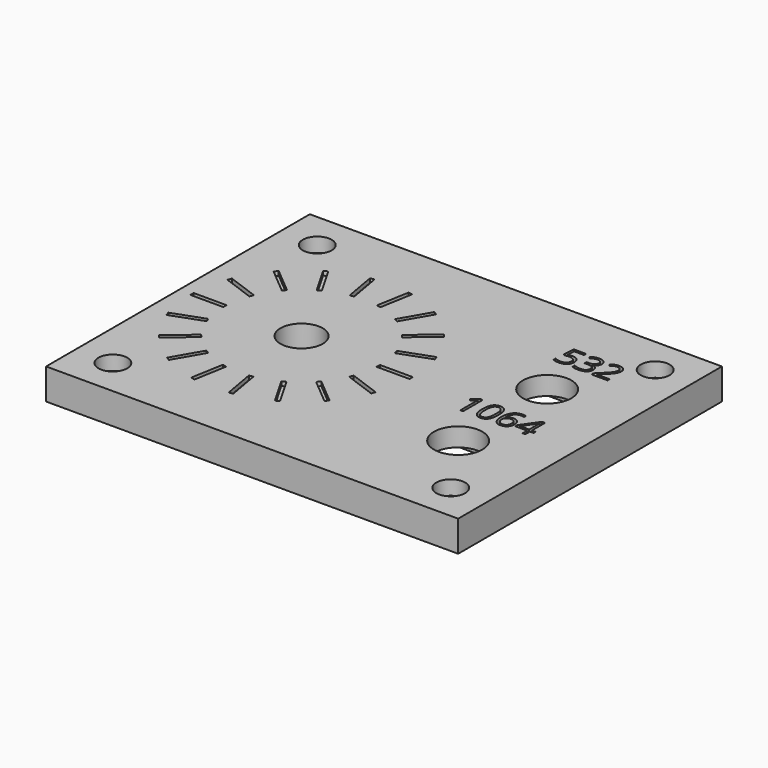
from build123d import *

# Parameters (mm, degrees)
F0_W          = 100
F0_H          = 80
F1_DEPTH      = 6
F2_R          = 5.125
F3_DEPTH      = 25
F4_W          = 8
F4_H          = 1
F5_DEPTH      = 1
F6_R          = 5.875
F7_DEPTH      = 6.001
F8_W          = 25
F8_H          = 14
F9_DEPTH      = 1.5
F10_R         = 3.5
F11_DEPTH     = 3.5
F12_R         = 2.375
F13_DEPTH     = 6.001
F14_TEXT_SIZE = 8.3333333333
F15_DEPTH     = 1.5
F16_W         = 100
F16_H         = 80
F16_W_2       = 96
F16_H_2       = 76
F17_DEPTH     = 1.5
F18_W         = 4
F18_H         = 4
F19_DEPTH     = 3


# Not quite as in the source:
# - Text() gives the source's letters only with a copy of the font that has no kerning and outlines rounded to 1/6400 em; it was checked with that copy


with BuildPart() as f1:
    # F0 (on Top) → F1 (new body)
    with BuildSketch(Plane.XY):
        with Locations((50, 40)):
            Rectangle(F0_W, F0_H)
    extrude(amount=F1_DEPTH)

    # F2 (on face) → F3 (cut)
    with BuildSketch(Plane.XY.offset(6)):
        with Locations((30, 40)):
            Circle(F2_R)
    extrude(amount=-F3_DEPTH, mode=Mode.SUBTRACT)

    # F4 (on face) → F5 (cut)
    with BuildSketch(Plane.XY.offset(6)):
        with Locations((7, 40.5)):
            Rectangle(F4_W, F4_H)
        Polygon((4.6282992388, 30.7654561302), (12.1458402051, 33.5016172768), (11.8038200617, 34.4413098976), (4.2862790955, 31.705148751), align=None)
        Polygon((9.3168000358, 22.6447345385), (15.4451555807, 27.787035416), (14.8023679711, 28.5530798591), (8.6740124261, 23.4107789816), align=None)
        Polygon((16.5, 16.6173140978), (20.5, 23.5455173281), (19.6339745962, 24.0455173281), (15.6339745962, 17.1173140978), align=None)
        Polygon((25.311499203, 13.4101906687), (26.7006846243, 21.2886526928), (25.7158768713, 21.4623008704), (24.32669145, 13.5838388463), align=None)
        Polygon((34.688500797, 13.4101906687), (33.2993153757, 21.2886526928), (32.3145076227, 21.1150045151), (33.703693044, 13.236542491), align=None)
        Polygon((43.5, 16.6173140978), (39.5, 23.5455173281), (38.6339745962, 23.0455173281), (42.6339745962, 16.1173140978), align=None)
        Polygon((50.6831999642, 22.6447345385), (44.5548444193, 27.787035416), (43.9120568096, 27.0209909728), (50.0404123545, 21.8786900953), align=None)
        Polygon((55.3717007612, 30.7654561302), (47.8541597949, 33.5016172768), (47.5121396516, 32.561924656), (55.0296806179, 29.8257635094), align=None)
        with Locations((53, 39.5)):
            Rectangle(F4_W, F4_H)
        Polygon((55.3717007612, 49.2345438698), (47.8541597949, 46.4983827232), (48.1961799383, 45.5586901024), (55.7137209045, 48.294851249), align=None)
        Polygon((50.6831999642, 57.3552654615), (44.5548444193, 52.212964584), (45.1976320289, 51.4469201409), (51.3259875739, 56.5892210184), align=None)
        Polygon((43.5, 63.3826859022), (39.5, 56.4544826719), (40.3660254038, 55.9544826719), (44.3660254038, 62.8826859022), align=None)
        Polygon((34.688500797, 66.5898093313), (33.2993153757, 58.7113473072), (34.2841231287, 58.5376991296), (35.67330855, 66.4161611537), align=None)
        Polygon((25.311499203, 66.5898093313), (26.7006846243, 58.7113473072), (27.6854923773, 58.8849954849), (26.296306956, 66.763457509), align=None)
        Polygon((16.5, 63.3826859022), (20.5, 56.4544826719), (21.3660254038, 56.9544826719), (17.3660254038, 63.8826859022), align=None)
        Polygon((9.3168000358, 57.3552654615), (15.4451555807, 52.212964584), (16.0879431904, 52.9790090272), (9.9595876455, 58.1213099047), align=None)
        Polygon((4.6282992388, 49.2345438698), (12.1458402051, 46.4983827232), (12.4878603484, 47.438075344), (4.9703193821, 50.1742364906), align=None)
    extrude(amount=-F5_DEPTH, mode=Mode.SUBTRACT)

    # F6 (on face) → F7 (cut, through all)
    with BuildSketch(Plane.XY.offset(6)):
        with Locations((80, 25)):
            Circle(F6_R)
        with Locations((80, 52)):
            Circle(F6_R)
    extrude(amount=-F7_DEPTH, mode=Mode.SUBTRACT)

    # F8 (on face) → F9 (cut)
    with BuildSketch(Plane(origin=(0, 0, 0), x_dir=(1, 0, 0), z_dir=(0, 0, -1))):
        with Locations((80, -52)):
            Rectangle(F8_W, F8_H)
        with Locations((80, -25)):
            Rectangle(F8_W, F8_H)
    extrude(amount=-F9_DEPTH, mode=Mode.SUBTRACT)

    # F10 (on face) → F11 (cut)
    with BuildSketch(Plane.XY.offset(6)):
        with Locations((9, 9)):
            Circle(F10_R)
        with Locations((91, 9)):
            Circle(F10_R)
        with Locations((91, 71)):
            Circle(F10_R)
        with Locations((9, 71)):
            Circle(F10_R)
    extrude(amount=-F11_DEPTH, mode=Mode.SUBTRACT)

    # F12 (on face) → F13 (cut, through all)
    with BuildSketch(Plane.XY.offset(6)):
        with Locations((9, 71)):
            Circle(F12_R)
        with Locations((9, 9)):
            Circle(F12_R)
        with Locations((91, 9)):
            Circle(F12_R)
        with Locations((91, 71)):
            Circle(F12_R)
    extrude(amount=-F13_DEPTH, mode=Mode.SUBTRACT)

    # F14 (on face) → F15 (cut)
    with BuildSketch(Plane.XY.offset(6)):
        with Locations((72.806640625, 62)):
            Text('532', F14_TEXT_SIZE, font='Open Sans', text_align=(TextAlign.LEFT, TextAlign.BOTTOM))
        with Locations((70.2845052083, 35)):
            Text('1064', F14_TEXT_SIZE, font='Open Sans', text_align=(TextAlign.LEFT, TextAlign.BOTTOM))
    extrude(amount=-F15_DEPTH, mode=Mode.SUBTRACT)

    # F16 (on face) → F17 (join)
    with BuildSketch(Plane(origin=(0, 0, 0), x_dir=(1, 0, 0), z_dir=(0, 0, -1))):
        with Locations((50, -40)):
            Rectangle(F16_W, F16_H)
        with Locations((50, -40)):
            Rectangle(F16_W_2, F16_H_2, mode=Mode.SUBTRACT)
    extrude(amount=F17_DEPTH)

    # F18 (on face) → F19 (cut)
    with BuildSketch(Plane(origin=(0, 0, 0), x_dir=(1, 0, 0), z_dir=(0, 0, -1))):
        with Locations((18.5, -40)):
            Rectangle(F18_W, F18_H)
    extrude(amount=-F19_DEPTH, mode=Mode.SUBTRACT)


solid = f1.part
